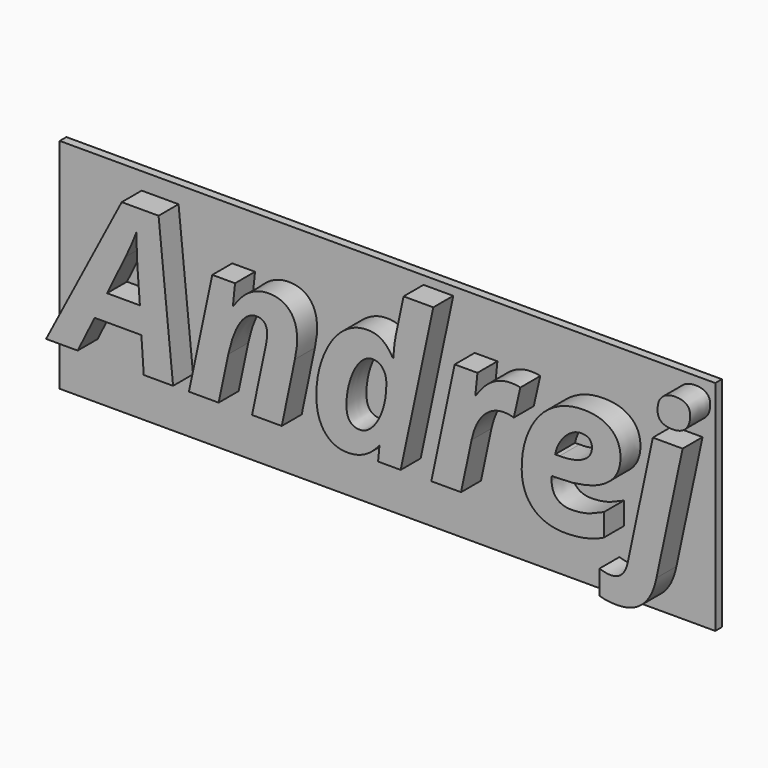
from build123d import *

# Parameters (mm, degrees)
F0_TEXT_SIZE = 24.314187174
F1_DEPTH     = 3
F2_W         = 78.7897594273
F2_H         = 26.2312022969
F3_DEPTH     = 1


# Not quite as in the source:
# - Text() gives the source's letters only with a copy of the font that has no kerning and outlines rounded to 1/6400 em; it was checked with that copy


with BuildPart() as f1:
    # F0 (on Front) → F1 (new body)
    with BuildSketch(Plane.XZ):
        with Locations((-44.7518088037, -0.1232831214)):
            Text('Andrej', F0_TEXT_SIZE, font='Open Sans', font_style=FontStyle.BOLDITALIC, text_align=(TextAlign.LEFT, TextAlign.BOTTOM))
    extrude(amount=F1_DEPTH)

    # F2 (on face) → F3 (join)
    with BuildSketch(Plane.XZ):
        with Locations((-7.575230673, 6.2478301115)):
            Rectangle(F2_W, F2_H)
    extrude(amount=-F3_DEPTH)


solid = f1.part
